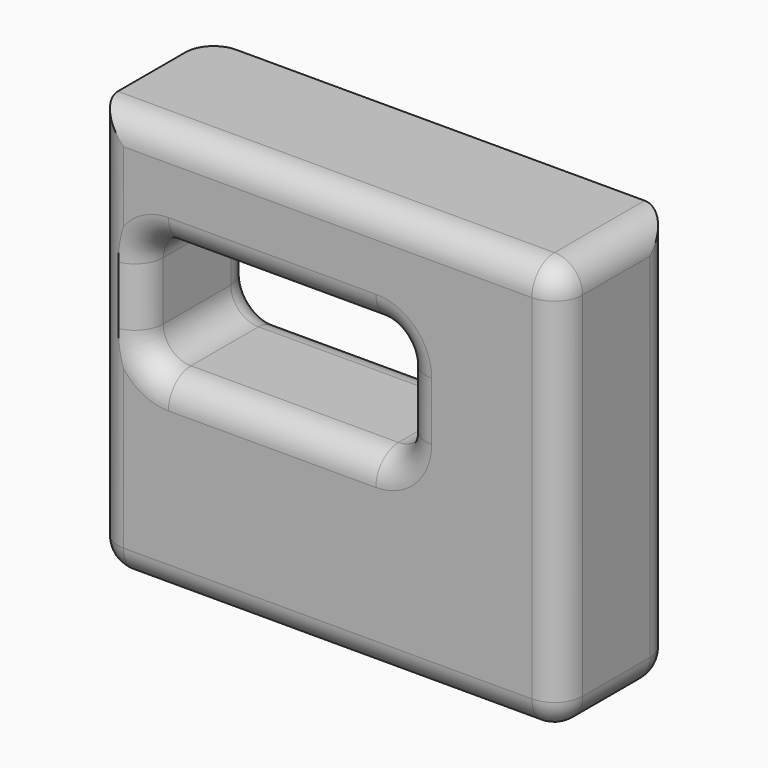
from build123d import *

# Parameters (mm, degrees)
F0_W         = 83.8200002909
F0_H         = 73.8754719496
F1_DEPTH     = 25.4
F3_DEPTH     = 25.4
F4_R         = 5.08
F5_T1_DEPTH  = 63.7154719496
F5_T3_DEPTH  = 73.6600002909
F5_T5_DEPTH  = 81.4954719496
F5_T7_DEPTH  = 37.4158525467
F5_T9_DEPTH  = 15.24
F5_T11_DEPTH = 10.5305814743
F5_T13_DEPTH = 91.4400002909
F5_S17_W     = 5.08
F5_S17_H     = 5.08
F5_T18_DEPTH = 5.08
F5_S23_W     = 5.08
F5_S23_H     = 5.08
F5_T24_DEPTH = 5.08
F5_S29_W     = 5.08
F5_S29_H     = 5.08
F5_T30_DEPTH = 5.08
F5_T34_ANGLE = 90
F5_T36_ANGLE = 90
F5_T38_ANGLE = 90
F5_T40_ANGLE = 90
F5_T42_ANGLE = 90
F5_T44_ANGLE = 90
F5_T46_ANGLE = 90
F5_T48_ANGLE = 90
F5_T50_ANGLE = 90
F5_T52_ANGLE = 90


# Not quite as in the source:
# - a fillet or chamfer that OpenCascade refuses, or shapes differently, is made with other operations: its cross-section is extruded or revolved along the edge and cut away or added
# - a feature names something its author has since deleted; it is built from what else it names


with BuildPart() as f1:
    # F0 (on Front) → F1 (new body)
    with BuildSketch(Plane.XZ):
        with Locations((-13.6877670884, 18.9792513847)):
            Rectangle(F0_W, F0_H)
    extrude(amount=F1_DEPTH)

    # F2 (on face) → F3 (cut)
    with BuildSketch(Plane.XZ.offset(25.4)):
        with BuildLine():
            ThreePointArc((0, 32.1505618095), (-1.4644660941, 35.6860957155), (-5, 37.1505618095))
            Line((-5, 37.1505618095), (-42.4158525467, 37.1505618095))
            ThreePointArc((-42.4158525467, 37.1505618095), (-45.9513864526, 35.6860957155), (-47.4158525467, 32.1505618095))
            Line((-47.4158525467, 32.1505618095), (-47.4158525467, 21.6199803352))
            ThreePointArc((-47.4158525467, 21.6199803352), (-45.9513864526, 18.0844464293), (-42.4158525467, 16.6199803352))
            Line((-42.4158525467, 16.6199803352), (-5, 16.6199803352))
            ThreePointArc((-5, 16.6199803352), (-1.4644660941, 18.0844464293), (0, 21.6199803352))
            Line((0, 21.6199803352), (0, 32.1505618095))
        make_face()
    extrude(amount=-F3_DEPTH, mode=Mode.SUBTRACT)

    # F4
    f4_edges = [f1.edges().sort_by_distance(p)[0] for p in [
        (28.222233, 0, 18.979251),
        (28.222233, -12.7, 55.916987),
    ]]
    fillet(f4_edges, radius=F4_R)

    # F5: fillet of radius 5.08 on 10 edges, made by hand

    # F5_s2 → F5_t1 (cut)
    with BuildSketch(Plane.XY.offset(-12.8784845901)):
        with BuildLine():
            ThreePointArc((23.142233057, -25.4), (26.7343355054, -23.9121024484), (28.222233057, -20.32))
            Line((28.222233057, -20.32), (28.222233057, -25.4))
            Line((28.222233057, -25.4), (23.142233057, -25.4))
        make_face()
    extrude(amount=F5_T1_DEPTH, mode=Mode.SUBTRACT)

    # F5_s4 → F5_t3 (cut)
    with BuildSketch(Plane.YZ.offset(-50.5177672338)):
        with BuildLine():
            ThreePointArc((-25.4, -12.8784845901), (-23.9121024484, -16.4705870385), (-20.32, -17.9584845901))
            Line((-20.32, -17.9584845901), (-25.4, -17.9584845901))
            Line((-25.4, -17.9584845901), (-25.4, -12.8784845901))
        make_face()
        with BuildLine():
            ThreePointArc((0, -12.8784845901), (-1.4878975516, -16.4705870385), (-5.08, -17.9584845901))
            Line((-5.08, -17.9584845901), (0, -17.9584845901))
            Line((0, -17.9584845901), (0, -12.8784845901))
        make_face()
    extrude(amount=F5_T3_DEPTH, mode=Mode.SUBTRACT)

    # F5_s6 → F5_t5 (cut)
    with BuildSketch(Plane.XY.offset(-12.8784845901)):
        with BuildLine():
            ThreePointArc((-55.5977672338, -20.32), (-54.1098696823, -23.9121024484), (-50.5177672338, -25.4))
            Line((-50.5177672338, -25.4), (-55.5977672338, -25.4))
            Line((-55.5977672338, -25.4), (-55.5977672338, -20.32))
        make_face()
        with BuildLine():
            ThreePointArc((-50.5177672338, 0), (-54.1098696823, -1.4878975516), (-55.5977672338, -5.08))
            Line((-55.5977672338, -5.08), (-55.5977672338, 0))
            Line((-55.5977672338, 0), (-50.5177672338, 0))
        make_face()
    extrude(amount=F5_T5_DEPTH, mode=Mode.SUBTRACT)

    # F5_s8 → F5_t7 (cut)
    with BuildSketch(Plane.YZ.offset(-42.4158525467)):
        with BuildLine():
            ThreePointArc((-25.4, 42.2305618095), (-23.9121024484, 38.6384593611), (-20.32, 37.1505618095))
            Line((-20.32, 37.1505618095), (-25.4, 37.1505618095))
            Line((-25.4, 37.1505618095), (-25.4, 42.2305618095))
        make_face()
        with BuildLine():
            ThreePointArc((0, 11.5399803352), (-1.4878975516, 15.1320827837), (-5.08, 16.6199803352))
            Line((-5.08, 16.6199803352), (0, 16.6199803352))
            Line((0, 16.6199803352), (0, 11.5399803352))
        make_face()
        with BuildLine():
            ThreePointArc((0, 42.2305618095), (-1.4878975516, 38.6384593611), (-5.08, 37.1505618095))
            Line((-5.08, 37.1505618095), (0, 37.1505618095))
            Line((0, 37.1505618095), (0, 42.2305618095))
        make_face()
        with BuildLine():
            ThreePointArc((-25.4, 11.5399803352), (-23.9121024484, 15.1320827837), (-20.32, 16.6199803352))
            Line((-20.32, 16.6199803352), (-25.4, 16.6199803352))
            Line((-25.4, 16.6199803352), (-25.4, 11.5399803352))
        make_face()
    extrude(amount=F5_T7_DEPTH, mode=Mode.SUBTRACT)

    # F5_s10 → F5_t9 (cut)
    with BuildSketch(Plane.XZ.offset(5.08)):
        with BuildLine():
            ThreePointArc((-55.5977672338, -12.8784845901), (-54.1098696823, -16.4705870385), (-50.5177672338, -17.9584845901))
            Line((-50.5177672338, -17.9584845901), (-55.5977672338, -17.9584845901))
            Line((-55.5977672338, -17.9584845901), (-55.5977672338, -12.8784845901))
        make_face()
        with BuildLine():
            ThreePointArc((23.142233057, -17.9584845901), (26.7343355054, -16.4705870385), (28.222233057, -12.8784845901))
            Line((28.222233057, -12.8784845901), (28.222233057, -17.9584845901))
            Line((28.222233057, -17.9584845901), (23.142233057, -17.9584845901))
        make_face()
    extrude(amount=F5_T9_DEPTH, mode=Mode.SUBTRACT)

    # F5_s12 → F5_t11 (cut)
    with BuildSketch(Plane.XY.offset(21.6199803352)):
        with BuildLine():
            ThreePointArc((-52.4958525467, 0), (-48.9037500983, -1.4878975516), (-47.4158525467, -5.08))
            Line((-47.4158525467, -5.08), (-47.4158525467, 0))
            Line((-47.4158525467, 0), (-52.4958525467, 0))
        make_face()
        with BuildLine():
            ThreePointArc((5.08, 0), (1.4878975516, -1.4878975516), (0, -5.08))
            Line((0, -5.08), (0, 0))
            Line((0, 0), (5.08, 0))
        make_face()
        with BuildLine():
            ThreePointArc((5.08, -25.4), (1.4878975516, -23.9121024484), (0, -20.32))
            Line((0, -20.32), (0, -25.4))
            Line((0, -25.4), (5.08, -25.4))
        make_face()
        with BuildLine():
            ThreePointArc((-52.4958525467, -25.4), (-48.9037500983, -23.9121024484), (-47.4158525467, -20.32))
            Line((-47.4158525467, -20.32), (-47.4158525467, -25.4))
            Line((-47.4158525467, -25.4), (-52.4958525467, -25.4))
        make_face()
    extrude(amount=F5_T11_DEPTH, mode=Mode.SUBTRACT)

    # F5_s14 → F5_t13 (cut)
    with BuildSketch(Plane.YZ.offset(-68.2977672338)):
        with BuildLine():
            ThreePointArc((-20.32, 55.9169873595), (-23.9121024484, 54.429089808), (-25.4, 50.8369873595))
            Line((-25.4, 50.8369873595), (-25.4, 55.9169873595))
            Line((-25.4, 55.9169873595), (-20.32, 55.9169873595))
        make_face()
    extrude(amount=F5_T13_DEPTH, mode=Mode.SUBTRACT)


with BuildPart() as f5_tool16:
    # F5_s17 → F5_t18 (new body)
    with BuildSketch(Plane.XZ.offset(20.32)):
        with Locations((25.682233057, -15.4184845901)):
            Rectangle(F5_S17_W, F5_S17_H)
    extrude(amount=F5_T18_DEPTH)

    # F5_s19 → F5_t20 (revolve, cut)
    with BuildSketch(Plane(origin=(23.142233057, -20.32, -12.8784845901), x_dir=(-0.7071067812, 0, 0.7071067812), z_dir=(0.7071067812, 0, 0.7071067812))):
        with BuildLine():
            ThreePointArc((0, -5.08), (5.08, 0), (0, 5.08))
            Line((0, 5.08), (0, -5.08))
        make_face()
    revolve(axis=Axis((23.142233057, -20.32, -12.8784845901), (0, -1, 0)), mode=Mode.SUBTRACT)


with BuildPart() as f1_1:
    add(f1.part)

    # F5_t15: cut F5_tool16
    add(f5_tool16.part, mode=Mode.SUBTRACT)


with BuildPart() as f5_tool22:
    # F5_s23 → F5_t24 (new body)
    with BuildSketch(Plane.YZ.offset(-50.5177672338)):
        with Locations((-22.86, -15.4184845901)):
            Rectangle(F5_S23_W, F5_S23_H)
    extrude(amount=-F5_T24_DEPTH)

    # F5_s25 → F5_t26 (revolve, cut)
    with BuildSketch(Plane(origin=(-50.5177672338, -20.32, -12.8784845901), x_dir=(0, 0.7071067812, 0.7071067812), z_dir=(0, -0.7071067812, 0.7071067812))):
        with BuildLine():
            ThreePointArc((0, -5.08), (5.08, 0), (0, 5.08))
            Line((0, 5.08), (0, -5.08))
        make_face()
    revolve(axis=Axis((-50.5177672338, -20.32, -12.8784845901), (-1, 0, 0)), mode=Mode.SUBTRACT)


with BuildPart() as f1_2:
    add(f1_1.part)

    # F5_t21: cut F5_tool22
    add(f5_tool22.part, mode=Mode.SUBTRACT)


with BuildPart() as f5_tool28:
    # F5_s29 → F5_t30 (new body)
    with BuildSketch(Plane.XZ.offset(5.08)):
        with Locations((-53.0577672338, -15.4184845901)):
            Rectangle(F5_S29_W, F5_S29_H)
    extrude(amount=-F5_T30_DEPTH)

    # F5_s31 → F5_t32 (revolve, cut)
    with BuildSketch(Plane(origin=(-50.5177672338, -5.08, -12.8784845901), x_dir=(0.7071067812, 0, 0.7071067812), z_dir=(-0.7071067812, 0, 0.7071067812))):
        with BuildLine():
            ThreePointArc((0, -5.08), (5.08, 0), (0, 5.08))
            Line((0, 5.08), (0, -5.08))
        make_face()
    revolve(axis=Axis((-50.5177672338, -5.08, -12.8784845901), (0, 1, 0)), mode=Mode.SUBTRACT)


with BuildPart() as f1_3:
    add(f1_2.part)

    # F5_t27: cut F5_tool28
    add(f5_tool28.part, mode=Mode.SUBTRACT)

    # F5_s33 → F5_t34 (revolve, cut)
    with BuildSketch(Plane.XY.offset(32.1505618095)):
        with BuildLine():
            ThreePointArc((5.08, -25.4), (1.4878975516, -23.9121024484), (0, -20.32))
            Line((0, -20.32), (0, -25.4))
            Line((0, -25.4), (5.08, -25.4))
        make_face()
    revolve(axis=Axis((-5, -25.4, 32.1505618095), (0, -1, 0)), revolution_arc=F5_T34_ANGLE, mode=Mode.SUBTRACT)

    # F5_s35 → F5_t36 (revolve, cut)
    with BuildSketch(Plane.XY.offset(21.6199803352)):
        with BuildLine():
            ThreePointArc((-52.4958525467, 0), (-48.9037500983, -1.4878975516), (-47.4158525467, -5.08))
            Line((-47.4158525467, -5.08), (-47.4158525467, 0))
            Line((-47.4158525467, 0), (-52.4958525467, 0))
        make_face()
    revolve(axis=Axis((-42.4158525467, 0, 21.6199803352), (0, -1, 0)), revolution_arc=F5_T36_ANGLE, mode=Mode.SUBTRACT)

    # F5_s37 → F5_t38 (revolve, cut)
    with BuildSketch(Plane.YZ.offset(-42.4158525467)):
        with BuildLine():
            ThreePointArc((0, 42.2305618095), (-1.4878975516, 38.6384593611), (-5.08, 37.1505618095))
            Line((-5.08, 37.1505618095), (0, 37.1505618095))
            Line((0, 37.1505618095), (0, 42.2305618095))
        make_face()
    revolve(axis=Axis((-42.4158525467, 0, 32.1505618095), (0, -1, 0)), revolution_arc=F5_T38_ANGLE, mode=Mode.SUBTRACT)

    # F5_s39 → F5_t40 (revolve, cut)
    with BuildSketch(Plane.XY.offset(32.1505618095)):
        with BuildLine():
            ThreePointArc((5.08, 0), (1.4878975516, -1.4878975516), (0, -5.08))
            Line((0, -5.08), (0, 0))
            Line((0, 0), (5.08, 0))
        make_face()
    revolve(axis=Axis((-5, 0, 32.1505618095), (0, -1, 0)), revolution_arc=F5_T40_ANGLE, mode=Mode.SUBTRACT)

    # F5_s41 → F5_t42 (revolve, cut)
    with BuildSketch(Plane.YZ.offset(-5)):
        with BuildLine():
            ThreePointArc((0, 11.5399803352), (-1.4878975516, 15.1320827837), (-5.08, 16.6199803352))
            Line((-5.08, 16.6199803352), (0, 16.6199803352))
            Line((0, 16.6199803352), (0, 11.5399803352))
        make_face()
    revolve(axis=Axis((-5, 0, 21.6199803352), (0, -1, 0)), revolution_arc=F5_T42_ANGLE, mode=Mode.SUBTRACT)

    # F5_s43 → F5_t44 (revolve, cut)
    with BuildSketch(Plane.XZ.offset(5.08)):
        with BuildLine():
            ThreePointArc((28.222233057, -12.8784845901), (26.7343355054, -16.4705870385), (23.142233057, -17.9584845901))
            Line((23.142233057, -17.9584845901), (28.222233057, -17.9584845901))
            Line((28.222233057, -17.9584845901), (28.222233057, -12.8784845901))
        make_face()
    revolve(axis=Axis((23.142233057, -5.08, -17.9584845901), (0, 0, 1)), revolution_arc=F5_T44_ANGLE, mode=Mode.SUBTRACT)

    # F5_s45 → F5_t46 (revolve, cut)
    with BuildSketch(Plane.YZ.offset(-5)):
        with BuildLine():
            ThreePointArc((-25.4, 11.5399803352), (-23.9121024484, 15.1320827837), (-20.32, 16.6199803352))
            Line((-20.32, 16.6199803352), (-25.4, 16.6199803352))
            Line((-25.4, 16.6199803352), (-25.4, 11.5399803352))
        make_face()
    revolve(axis=Axis((-5, -25.4, 21.6199803352), (0, -1, 0)), revolution_arc=F5_T46_ANGLE, mode=Mode.SUBTRACT)

    # F5_s47 → F5_t48 (revolve, cut)
    with BuildSketch(Plane.XY.offset(21.6199803352)):
        with BuildLine():
            ThreePointArc((-52.4958525467, -25.4), (-48.9037500983, -23.9121024484), (-47.4158525467, -20.32))
            Line((-47.4158525467, -20.32), (-47.4158525467, -25.4))
            Line((-47.4158525467, -25.4), (-52.4958525467, -25.4))
        make_face()
    revolve(axis=Axis((-42.4158525467, -25.4, 21.6199803352), (0, -1, 0)), revolution_arc=F5_T48_ANGLE, mode=Mode.SUBTRACT)

    # F5_s49 → F5_t50 (revolve, cut)
    with BuildSketch(Plane.YZ.offset(-42.4158525467)):
        with BuildLine():
            ThreePointArc((-25.4, 42.2305618095), (-23.9121024484, 38.6384593611), (-20.32, 37.1505618095))
            Line((-20.32, 37.1505618095), (-25.4, 37.1505618095))
            Line((-25.4, 37.1505618095), (-25.4, 42.2305618095))
        make_face()
    revolve(axis=Axis((-42.4158525467, -25.4, 32.1505618095), (0, -1, 0)), revolution_arc=F5_T50_ANGLE, mode=Mode.SUBTRACT)

    # F5_s51 → F5_t52 (revolve, cut)
    with BuildSketch(Plane.YZ.offset(23.142233057)):
        with BuildLine():
            ThreePointArc((-20.32, 55.9169873595), (-23.9121024484, 54.429089808), (-25.4, 50.8369873595))
            Line((-25.4, 50.8369873595), (-25.4, 55.9169873595))
            Line((-25.4, 55.9169873595), (-20.32, 55.9169873595))
        make_face()
    revolve(axis=Axis((23.142233057, -25.4, 50.8369873595), (0, 1, 0)), revolution_arc=F5_T52_ANGLE, mode=Mode.SUBTRACT)


solid = f1_3.part
